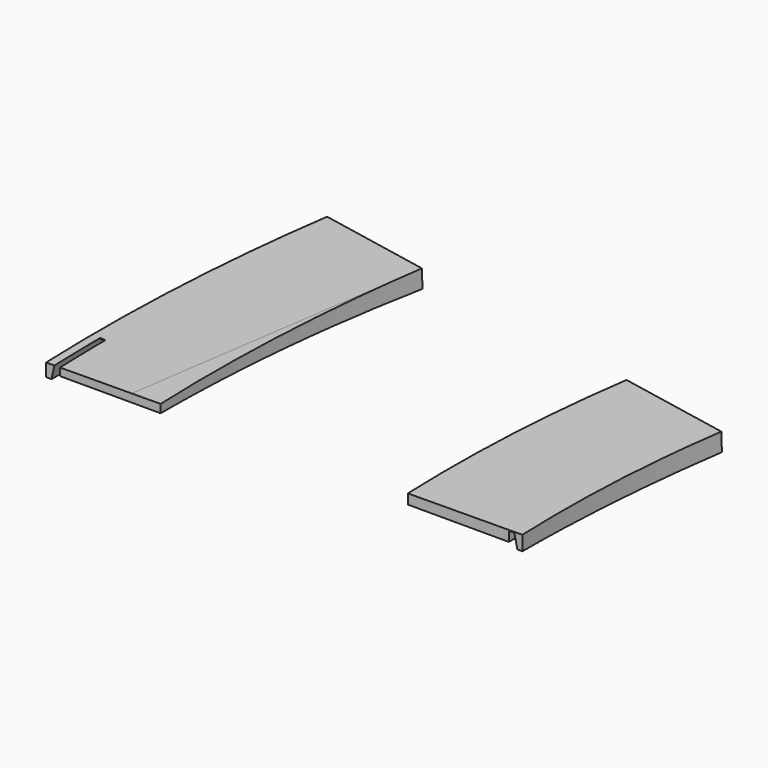
from build123d import *

# Parameters (mm, degrees)
F1_ANGLE_BACK = 11.25
F1_ANGLE      = 22.5
F2_W          = 148
F2_H          = 20.6737495929
F5_DEPTH      = 211.4
F7_DEPTH      = 234.2
F8_W          = 286.8234440684
F8_H          = 99.4558036327
F9_DEPTH      = 112
F11_ANGLE     = 30
F13_ANGLE     = 2


# Not quite as in the source:
# - a feature names something its author has since deleted; it is built from what else it names


with BuildPart() as f1:
    # F0 (on Front) → F1 (revolve)
    with BuildSketch(Plane.XZ, mode=Mode.PRIVATE) as f1_sk:
        Polygon((37.433034228, -1.662807624), (-0.066965772, -1.7883691504), (0, -21.7882570398), (37.5, -21.6626955134), align=None)
    revolve(f1_sk.sketch.rotate(Axis((525.8388087714, 0, 45.6422517605), (-0.1769446249, 0, 0.9842208084)), -F1_ANGLE_BACK), axis=Axis((525.8388087714, 0, 45.6422517605), (-0.1769446249, 0, 0.9842208084)), revolution_arc=F1_ANGLE)


with BuildPart() as f1b:
    # F0 (on Front) → F1, piece 2 (revolve)
    with BuildSketch(Plane.XZ, mode=Mode.PRIVATE) as f1_sk:
        Polygon((155.9321597647, -1.2660361285), (118.4321597647, -1.391597655), (118.4991255367, -21.3914855443), (155.9991255367, -21.2659240179), align=None)
    revolve(f1_sk.sketch.rotate(Axis((525.8388087714, 0, 45.6422517605), (-0.1769446249, 0, 0.9842208084)), -F1_ANGLE_BACK), axis=Axis((525.8388087714, 0, 45.6422517605), (-0.1769446249, 0, 0.9842208084)), revolution_arc=F1_ANGLE)


with BuildPart() as f3_tool:
    # F2 (on Front) → F3 (revolve)
    with BuildSketch(Plane.XZ):
        with Locations((78, -17.1368747965)):
            Rectangle(F2_W, F2_H)
    revolve(axis=Axis((526, 0, -40.4653474689), (0, 0, -1)))


with BuildPart() as f1_1:
    add(f1.part)

    # F3: cut by f3_tool
    add(f3_tool.part, mode=Mode.SUBTRACT)

    # F6 (on face) → F7 (cut)
    with BuildSketch(Plane(origin=(19.6894657776, 100.5725829361, 3.539800323), x_dir=(-0.9813925868, 0.1918931334, 0.0067539617), z_dir=(0.1920119545, 0.9807852804, 0.0345201838))):
        Polygon((9.9895421705, -4.4095212135), (35.8401375413, -4.5842232545), (37.4985628908, 20.4695294659), (-71.4865817421, 21.206066746), (-71.6559666141, -3.8577491241), (-27.5098117032, -4.1560951874), (-27.5044053117, -3.3561134558), (9.9949485621, -3.6095394819), align=None)
        Polygon((-27.5098117032, -4.1560951874), (9.9895421705, -4.4095212135), (9.9949485621, -3.6095394819), (-27.5044053117, -3.3561134558), align=None)
    extrude(amount=-F7_DEPTH, mode=Mode.SUBTRACT)


with BuildPart() as f1b_1:
    add(f1b.part)

    # F3: cut by f3_tool
    add(f3_tool.part, mode=Mode.SUBTRACT)

    # F4 (on face) → F5 (cut)
    with BuildSketch(Plane(origin=(19.6894657776, 100.5725829361, 3.539800323), x_dir=(-0.9813925868, 0.1918931334, 0.0067539617), z_dir=(0.1920119545, 0.9807852804, 0.0345201838))):
        Polygon((-108.5075416222, -3.6087008807), (-101.6713570142, -3.6549007994), (-102.5302484632, 6.0979337431), (-179.1422963142, 8.3114448935), (-179.1422963142, -3.1313410508), (-146.006895496, -3.3552748546), (-146.0014891044, -2.555293123), (-108.5021352307, -2.8087191491), align=None)
        Polygon((-146.006895496, -3.3552748546), (-108.5075416222, -3.6087008807), (-108.5021352307, -2.8087191491), (-146.0014891044, -2.555293123), align=None)
    extrude(amount=-F5_DEPTH, mode=Mode.SUBTRACT)


with BuildPart() as f9_tool:
    # F8 (on Front) → F9 (new body)
    with BuildSketch(Plane.XZ):
        with Locations((59.2738725245, -18.6479687691)):
            Rectangle(F8_W, F8_H)
    extrude(amount=F9_DEPTH)


with BuildPart() as f1_2:
    add(f1_1.part)

    # F9: cut by f9_tool
    add(f9_tool.part, mode=Mode.SUBTRACT)


with BuildPart() as f1b_2:
    add(f1b_1.part)

    # F9: cut by f9_tool
    add(f9_tool.part, mode=Mode.SUBTRACT)


with BuildPart() as f11_tool:
    # F10 (on Front) → F11 (revolve)
    with BuildSketch(Plane.XZ):
        Polygon((1.7227589607, -8.5826770598), (0.0227684901, -8.5883691504), (0.066965772, -21.7882570398), (4.5820021559, -21.7731393102), (4.5227488708, -4.0766501403), (2.7227589607, -4.0826770598), align=None)
        Polygon((156.0660913087, -21.2659240179), (156.0218940268, -8.0660361285), (154.3219035562, -8.0717282192), (153.3219035562, -3.5717282192), (151.5219136462, -3.5777551387), (151.5811893534, -21.2809408481), align=None)
        Polygon((0.066965772, -21.7882570398), (0.0227684901, -8.5883691504), (-1.582706409, -8.2315969506), (-1.532864623, -23.1172631943), align=None)
    revolve(axis=Axis((525.9057745435, 0, 45.6422517605), (0.1769446249, 0, -0.9842208084)), revolution_arc=F11_ANGLE)


with BuildPart() as f1_3:
    add(f1_2.part)

    # F11: cut by f11_tool
    add(f11_tool.part, mode=Mode.SUBTRACT)

    # F12 (on Front) → F13 (revolve, cut)
    with BuildSketch(Plane.XZ):
        Polygon((4.5227488708, -4.0766501403), (4.5227488708, -1.773225597), (2.7150464738, -1.7792783403), (2.7227589607, -4.0826770598), align=None)
    revolve(axis=Axis((525.9057745435, 0, 45.6422517605), (0.1769446249, 0, -0.9842208084)), revolution_arc=F13_ANGLE, mode=Mode.SUBTRACT)


with BuildPart() as f1b_3:
    add(f1b_2.part)

    # F11: cut by f11_tool
    add(f11_tool.part, mode=Mode.SUBTRACT)


solid = Compound([f1_3.part, f1b_3.part])
